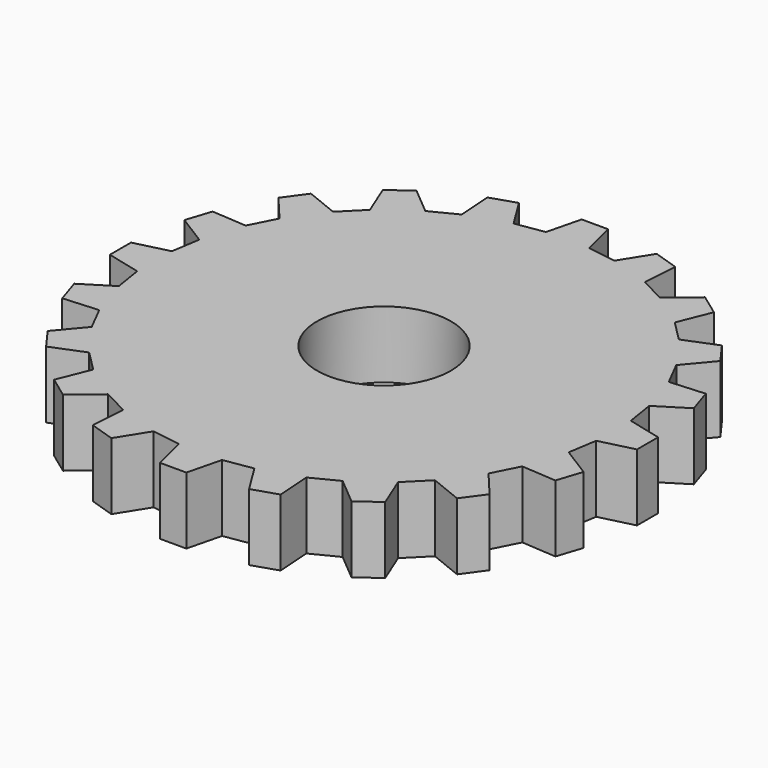
from build123d import *

# Parameters (mm, degrees)
F0_R     = 12.7
F1_DEPTH = 6.35


# Not quite as in the source:
# - a feature of the source that left no trace in its solid (it failed there, or was rolled back) is left out


with BuildPart() as f1:
    # F0 (on Top) → F1 (new body, symmetric)
    with BuildSketch(Plane.XY):
        Polygon((4.1113441396, 43.5372516477), (2.5, 50), (-2.5, 50), (-4.1113441396, 43.5372516477), (-9.5436300128, 42.6768620899), (-13.073208428, 48.3253683007), (-17.8284910095, 46.7802833288), (-17.3638712822, 40.1359116722), (-22.2644071652, 37.6389639237), (-27.3667201287, 41.9203128495), (-31.4118051006, 38.981386588), (-28.9167017225, 32.805789019), (-32.805789019, 28.9167017225), (-38.981386588, 31.4118051006), (-41.9203128495, 27.3667201287), (-37.6389639237, 22.2644071652), (-40.1359116722, 17.3638712822), (-46.7802833288, 17.8284910095), (-48.3253683007, 13.073208428), (-42.6768620899, 9.5436300128), (-43.5372516477, 4.1113441396), (-50, 2.5), (-50, -2.5), (-43.5372516477, -4.1113441396), (-42.6768620899, -9.5436300128), (-48.3253683007, -13.073208428), (-46.7802833288, -17.8284910095), (-40.1359116722, -17.3638712822), (-37.6389639237, -22.2644071652), (-41.9203128495, -27.3667201287), (-38.981386588, -31.4118051006), (-32.805789019, -28.9167017225), (-28.9167017225, -32.805789019), (-31.4118051006, -38.981386588), (-27.3667201287, -41.9203128495), (-22.2644071652, -37.6389639237), (-17.3638712822, -40.1359116722), (-17.8284910095, -46.7802833288), (-13.073208428, -48.3253683007), (-9.5436300128, -42.6768620899), (-4.1113441396, -43.5372516477), (-2.5, -50), (2.5, -50), (4.1113441396, -43.5372516477), (9.5436300128, -42.6768620899), (13.073208428, -48.3253683007), (17.8284910095, -46.7802833288), (17.3638712822, -40.1359116722), (22.2644071652, -37.6389639237), (27.3667201287, -41.9203128495), (31.4118051006, -38.981386588), (28.9167017225, -32.805789019), (32.805789019, -28.9167017225), (38.981386588, -31.4118051006), (41.9203128495, -27.3667201287), (37.6389639237, -22.2644071652), (40.1359116722, -17.3638712822), (46.7802833288, -17.8284910095), (48.3253683007, -13.073208428), (42.6768620899, -9.5436300128), (43.5372516477, -4.1113441396), (50, -2.5), (50, 2.5), (43.5372516477, 4.1113441396), (42.6768620899, 9.5436300128), (48.3253683007, 13.073208428), (46.7802833288, 17.8284910095), (40.1359116722, 17.3638712822), (37.6389639237, 22.2644071652), (41.9203128495, 27.3667201287), (38.981386588, 31.4118051006), (32.805789019, 28.9167017225), (28.9167017225, 32.805789019), (31.4118051006, 38.981386588), (27.3667201287, 41.9203128495), (22.2644071652, 37.6389639237), (17.3638712822, 40.1359116722), (17.8284910095, 46.7802833288), (13.073208428, 48.3253683007), (9.5436300128, 42.6768620899), align=None)
        Circle(F0_R, mode=Mode.SUBTRACT)
    extrude(amount=F1_DEPTH, both=True)


solid = f1.part
